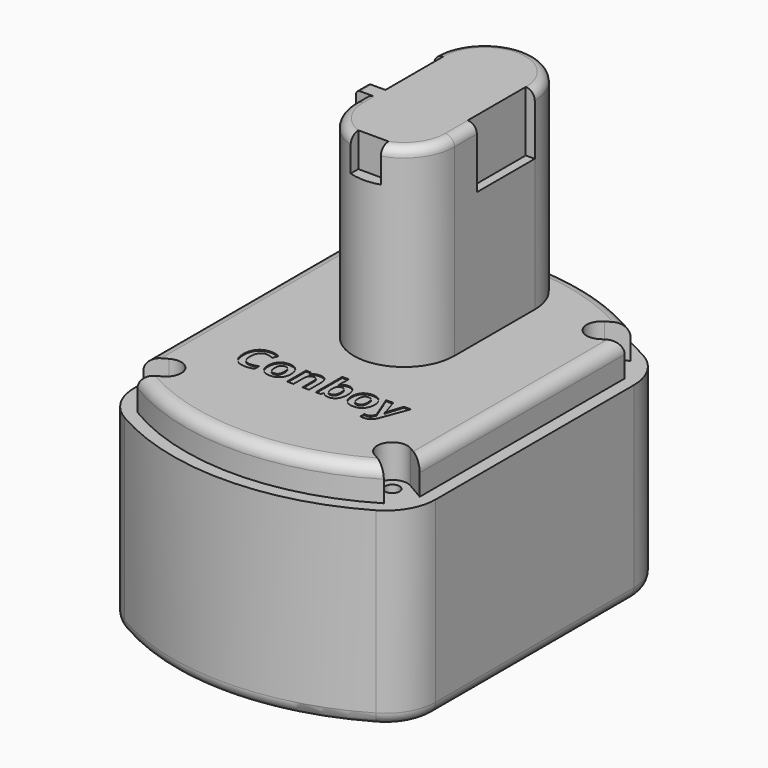
from build123d import *

# Parameters (mm, degrees)
F1_DEPTH      = 48.26
F3_DEPTH      = 8.382
F5_DEPTH      = 8.382
F6_R          = 1.8288
F7_DEPTH      = 32.8422
F9_DEPTH      = 57.15
F10_W         = 2.286
F10_H         = 3.556
F11_DEPTH     = 48.768
F12_R         = 2.286
F13_W         = 2.286
F13_H         = 18.288
F14_DEPTH     = 15.24
F16_DEPTH     = 8.636
F17_R         = 1.016
F18_TEXT_SIZE = 11.0419444444
F19_DEPTH     = 0.254
F20_R         = 12.7
F21_R         = 3.048
F22_R         = 3.175


# Not quite as in the source:
# - Text() gives the source's letters only with a copy of the font that has no kerning and outlines rounded to 1/6400 em; it was checked with that copy


with BuildPart() as f1:
    # F0 (on Top) → F1 (new body)
    with BuildSketch(Plane.XY):
        with BuildLine():
            Line((38.1, -38.1), (38.1, 38.1))
            ThreePointArc((38.1, 38.1), (0, 50.8), (-38.1, 38.1))
            Line((-38.1, 38.1), (-38.1, -38.1))
            ThreePointArc((-38.1, -38.1), (0, -50.8), (38.1, -38.1))
        make_face()
    extrude(amount=-F1_DEPTH)

    # F2 (on face) → F3 (join)
    with BuildSketch(Plane.XY):
        with BuildLine():
            Line((34.925, -36.4868884968), (34.925, 36.4868884968))
            ThreePointArc((34.925, 36.4868884968), (0, 47.625), (-34.925, 36.4868884968))
            Line((-34.925, 36.4868884968), (-34.925, -36.4868884968))
            ThreePointArc((-34.925, -36.4868884968), (0, -47.625), (34.925, -36.4868884968))
        make_face()
    extrude(amount=F3_DEPTH)

    # F4 (on face) → F5 (cut, through all)
    with BuildSketch(Plane.XY.offset(8.382)):
        with BuildLine():
            ThreePointArc((-26.67, -36.3957567884), (-25.2754432116, -31.1912), (-30.48, -29.7966432116))
            Line((-30.48, -29.7966432116), (-52.4770452561, -42.4966432116))
            ThreePointArc((-52.4770452561, -42.4966432116), (-53.8716020445, -47.7012), (-48.6670452561, -49.0957567884))
            Line((-48.6670452561, -49.0957567884), (-26.67, -36.3957567884))
        make_face()
        with BuildLine():
            ThreePointArc((30.48, -29.7966432116), (25.2754432116, -31.1912), (26.67, -36.3957567884))
            Line((26.67, -36.3957567884), (48.6670452561, -49.0957567884))
            ThreePointArc((48.6670452561, -49.0957567884), (53.8716020445, -47.7012), (52.4770452561, -42.4966432116))
            Line((52.4770452561, -42.4966432116), (30.48, -29.7966432116))
        make_face()
        with BuildLine():
            Line((-52.4770452561, 42.4966432116), (-30.48, 29.7966432116))
            ThreePointArc((-30.48, 29.7966432116), (-25.2754432116, 31.1912), (-26.67, 36.3957567884))
            Line((-26.67, 36.3957567884), (-48.6670452561, 49.0957567884))
            ThreePointArc((-48.6670452561, 49.0957567884), (-53.8716020445, 47.7012), (-52.4770452561, 42.4966432116))
        make_face()
        with BuildLine():
            ThreePointArc((26.67, 36.3957567884), (25.2754432116, 31.1912), (30.48, 29.7966432116))
            Line((30.48, 29.7966432116), (52.4770452561, 42.4966432116))
            ThreePointArc((52.4770452561, 42.4966432116), (53.8716020445, 47.7012), (48.6670452561, 49.0957567884))
            Line((48.6670452561, 49.0957567884), (26.67, 36.3957567884))
        make_face()
    extrude(amount=-F5_DEPTH, mode=Mode.SUBTRACT)

    # F6 (on face) → F7 (cut)
    with BuildSketch(Plane.XY):
        with Locations((-28.575, 33.0962)):
            Circle(F6_R)
        with Locations((28.575, 33.0962)):
            Circle(F6_R)
        with Locations((-28.575, -33.0962)):
            Circle(F6_R)
        with Locations((28.575, -33.0962)):
            Circle(F6_R)
    extrude(amount=-F7_DEPTH, mode=Mode.SUBTRACT)

    # F8 (on Top) → F9 (join)
    with BuildSketch(Plane.XY):
        with BuildLine():
            ThreePointArc((-12.7, 6.35), (0, -6.35), (12.7, 6.35))
            Line((12.7, 6.35), (12.7, 31.75))
            ThreePointArc((12.7, 31.75), (0, 44.45), (-12.7, 31.75))
            Line((-12.7, 31.75), (-12.7, 6.35))
        make_face()
    extrude(amount=F9_DEPTH)

    # F10 (on face) → F11 (join, through all)
    with BuildSketch(Plane.XY.offset(8.382)):
        with Locations((-13.843, 11.684)):
            Rectangle(F10_W, F10_H)
    extrude(amount=F11_DEPTH)

    # F12
    f12_edges = [f1.edges().sort_by_distance(p)[0] for p in [
        (12.7, 19.05, 57.15),
    ]]
    fillet(f12_edges, radius=F12_R)

    # F13 (on face) → F14 (cut)
    with BuildSketch(Plane.XY.offset(57.15)):
        with Locations((11.557, 22.606)):
            Rectangle(F13_W, F13_H)
        with Locations((-11.557, 22.606)):
            Rectangle(F13_W, F13_H)
    extrude(amount=-F14_DEPTH, mode=Mode.SUBTRACT)

    # F15 (on face) → F16 (cut)
    with BuildSketch(Plane.XY.offset(57.15)):
        with BuildLine():
            Line((-3.81, -3.3420222864), (-3.81, -5.765027858))
            ThreePointArc((-3.81, -5.765027858), (0, -6.35), (3.81, -5.765027858))
            Line((3.81, -5.765027858), (3.81, -3.3420222864))
            Line((3.81, -3.3420222864), (-3.81, -3.3420222864))
        make_face()
    extrude(amount=-F16_DEPTH, mode=Mode.SUBTRACT)

    # F17
    f17_edges = [f1.edges().sort_by_distance(p)[0] for p in [
        (-14.986, 11.684, 57.15),
    ]]
    fillet(f17_edges, radius=F17_R)

    # F18 (on face) → F19 (cut)
    with BuildSketch(Plane.XY.offset(8.382)):
        with Locations((-20.9762438368, -22.86)):
            Text('Conboy', F18_TEXT_SIZE, font='Open Sans', font_style=FontStyle.BOLD, text_align=(TextAlign.LEFT, TextAlign.BOTTOM))
    extrude(amount=-F19_DEPTH, mode=Mode.SUBTRACT)

    # F20
    f20_edges = [f1.edges().sort_by_distance(p)[0] for p in [
        (38.1, -38.1, -24.13),
        (38.1, 38.1, -24.13),
        (-38.1, -38.1, -24.13),
        (-38.1, 38.1, -24.13),
    ]]
    fillet(f20_edges, radius=F20_R)

    # F21
    f21_edges = [f1.edges().sort_by_distance(p)[0] for p in [
        (0, -47.625, 8.382),
        (34.925, 0, 8.382),
        (0, 47.625, 8.382),
        (-34.925, 0, 8.382),
    ]]
    fillet(f21_edges, radius=F21_R)

    # F22
    f22_edges = [f1.edges().sort_by_distance(p)[0] for p in [
        (38.1, 0, -48.26),
    ]]
    fillet(f22_edges, radius=F22_R)


solid = f1.part
